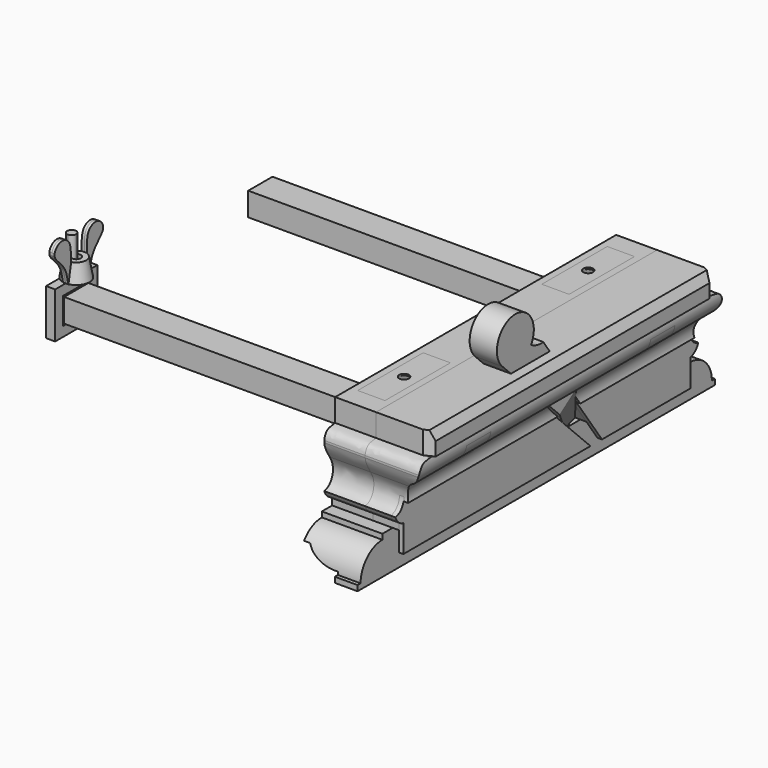
from build123d import *

# Parameters (mm, degrees)
F1_DEPTH  = 250
F2_DEPTH  = 250
F3_W      = 6.5
F3_H      = 13
F4_DEPTH  = 37.001
F8_DEPTH  = 15
F9_DEPTH  = 15
F10_W     = 20
F10_H     = 15.5
F11_DEPTH = 35.8337030046
F12_DEPTH = 50
F13_DEPTH = 230
F15_DEPTH = 20
F17_DEPTH = 20
F21_DEPTH = 9
F22_DEPTH = 27
F24_DEPTH = 40
F25_W     = 25
F25_H     = 3.6049708724
F26_DEPTH = 295.0010001
F27_DEPTH = 9
F29_REACH = 207.1008130873
F30_W     = 7
F30_H     = 35
F30_R     = 3.25
F31_DEPTH = 47
F30_W_2   = 18
F30_H_2   = 54
F32_DEPTH = 1
F33_DEPTH = 1
F34_DEPTH = 1
F35_W     = 22
F35_H     = 17.5
F36_DEPTH = 6
F37_R     = 2.99999
F39_DEPTH = 1.75


# Not quite as in the source:
# - a fillet or chamfer is up to 0.001 mm smaller than in the source, because OpenCascade refuses the exact size
# - a feature of the source that left no trace in its solid (it failed there, or was rolled back) is left out


with BuildPart() as f1:
    # F0 (on Front) → F1 (new body)
    with BuildSketch(Plane.XZ):
        with BuildLine():
            Line((0, 19.1666619313), (0, 0))
            Line((0, 0), (0, -42.8333380687))
            Line((0, -42.8333380687), (17, -42.8333380687))
            Line((17, -42.8333380687), (17, -22.8333380687))
            Line((17, -22.8333380687), (20, -22.8333380687))
            Line((20, -22.8333380687), (20, -25.2570672073))
            Line((20, -25.2570672073), (23, -25.2570672073))
            ThreePointArc((23, -25.2570672073), (23.5967218154, -16.8270536205), (29.25, -10.545202638))
            Line((29.25, -10.545202638), (35.5, 4.1666619313))
            Line((35.5, 4.1666619313), (37, 4.1666619313))
            Line((37, 4.1666619313), (37, 13.1666619313))
            Line((37, 13.1666619313), (34, 19.1666619313))
            Line((34, 19.1666619313), (0, 19.1666619313))
        make_face()
        with BuildLine():
            ThreePointArc((29.25, -10.545202638), (34.9032781846, -4.2633516555), (35.5, 4.1666619313))
            Line((35.5, 4.1666619313), (29.25, -10.545202638))
        make_face()
    extrude(amount=F1_DEPTH)


with BuildPart() as f2:
    # F0 (on Front) → F2 (new body)
    with BuildSketch(Plane.XZ):
        Polygon((17, -22.8333380687), (17, -42.8333380687), (17, -55.8333380687), (20, -55.8333380687), (20, -25.2570672073), (20, -22.8333380687), align=None)
    extrude(amount=F2_DEPTH)


with BuildPart() as f4_tool:
    # F3 (on face) → F4 (new body, through all)
    with BuildSketch(Plane(origin=(0, 0, 0), x_dir=(0, -1, 0), z_dir=(-1, 0, 0))):
        with BuildLine():
            Line((9, 4.1666619313), (9, 19.1666619313))
            Line((9, 19.1666619313), (0, 19.1666619313))
            Line((0, 19.1666619313), (0, -2.3163000296))
            add(Edge.make_bspline(
                [(9, 4.1666619313), (5.8723544835, 3.6611618628), (2.3380474739, 3.7477802491), (0.1732748267, -0.2324329033), (0, -2.3163000296)],
                knots=[0, 0, 0, 0, 0.1389392209, 0.2524518766, 0.2524518766, 0.2524518766, 0.2524518766], degree=3))
        make_face()
        with BuildLine():
            Line((250, 19.1666619313), (241, 19.1666619313))
            Line((241, 19.1666619313), (241, 4.1666619313))
            add(Edge.make_bspline(
                [(241, 4.1666619313), (244.1276455165, 3.6611618628), (247.6619525261, 3.7477802491), (249.8267251733, -0.2324329033), (250, -2.3163000296)],
                knots=[0, 0, 0, 0, 0.1389392209, 0.2524518766, 0.2524518766, 0.2524518766, 0.2524518766], degree=3))
            Line((250, -2.3163000296), (250, 19.1666619313))
        make_face()
        with BuildLine():
            add(Edge.make_bspline(
                [(4.5, -13.8333380687), (5.7822039131, -16.0114235416), (7.4274862503, -19.2486278619), (7.1721404656, -25.7962519699), (4.6179848399, -29.5292930366), (2.9422229886, -30.8853534567), (0.7419204277, -31.6729300915), (0, -31.8333380687)],
                knots=[0.4537350844, 0.4537350844, 0.4537350844, 0.4537350844, 0.5873526723, 0.7194908339, 0.8294393125, 0.9086679454, 1, 1, 1, 1], degree=3))
            Line((4.5, -13.8333380687), (0, -31.8333380687))
        make_face()
        with BuildLine():
            Line((0, -31.8333380687), (4.5, -13.8333380687))
            add(Edge.make_bspline(
                [(0, -3.6448843312), (0.283077162, -7.0636780394), (2.7941794565, -10.9356531472), (4.5, -13.8333380687)],
                knots=[0.2759726988, 0.2759726988, 0.2759726988, 0.2759726988, 0.4537350844, 0.4537350844, 0.4537350844, 0.4537350844], degree=3))
            Line((0, -3.6448843311), (0, -31.8333380687))
        make_face()
        with BuildLine():
            ThreePointArc((6.5, -37.8333380687), (2.4506727422, -35.6992759313), (0, -31.8333380687))
            Line((0, -31.8333380687), (0, -42.8333380687))
            Line((0, -42.8333380687), (6.5, -42.8333380687))
            Line((6.5, -42.8333380687), (6.5, -37.8333380687))
        make_face()
        with BuildLine():
            Line((250, -31.8333380687), (245.5, -13.8333380687))
            add(Edge.make_bspline(
                [(245.5, -13.8333380687), (244.2177960869, -16.0114235416), (242.5725137497, -19.2486278619), (242.8278595344, -25.7962519699), (245.3820151601, -29.5292930366), (247.0577770114, -30.8853534567), (249.2580795723, -31.6729300915), (250, -31.8333380687)],
                knots=[0.4537350844, 0.4537350844, 0.4537350844, 0.4537350844, 0.5873526723, 0.7194908339, 0.8294393125, 0.9086679454, 1, 1, 1, 1], degree=3))
        make_face()
        with BuildLine():
            add(Edge.make_bspline(
                [(250, -3.6448843312), (249.716922838, -7.0636780394), (247.2058205435, -10.9356531472), (245.5, -13.8333380687)],
                knots=[0.2759726988, 0.2759726988, 0.2759726988, 0.2759726988, 0.4537350844, 0.4537350844, 0.4537350844, 0.4537350844], degree=3))
            Line((245.5, -13.8333380687), (250, -31.8333380687))
            Line((250, -31.8333380687), (250, -3.6448843312))
        make_face()
        with Locations((3.25, -49.3333380687)):
            Rectangle(F3_W, F3_H)
        with BuildLine():
            Line((250, -42.8333380687), (250, -31.8333380687))
            ThreePointArc((250, -31.8333380687), (247.5493272578, -35.6992759313), (243.5, -37.8333380687))
            Line((243.5, -37.8333380687), (243.5, -42.8333380687))
            Line((243.5, -42.8333380687), (250, -42.8333380687))
        make_face()
        with Locations((246.75, -49.3333380687)):
            Rectangle(F3_W, F3_H)
    extrude(amount=-F4_DEPTH)


with BuildPart() as f1_1:
    add(f1.part)

    # F4: cut by f4_tool
    add(f4_tool.part, mode=Mode.SUBTRACT)

    # F7 (on face) → F8 (cut, through all)
    with BuildSketch(Plane.XY.offset(19.1666619313)):
        Polygon((34, -10.5), (34, -9), (31, -9), align=None)
        Polygon((37, -9), (34, -9), (34, -10.5), (37, -12), align=None)
    extrude(amount=-F8_DEPTH, mode=Mode.SUBTRACT)

    # F7 (on face) → F9 (cut, through all)
    with BuildSketch(Plane.XY.offset(19.1666619313)):
        Polygon((37, -238), (34, -239.5), (34, -241), (37, -241), align=None)
        Polygon((34, -241), (34, -239.5), (31, -241), align=None)
    extrude(amount=-F9_DEPTH, mode=Mode.SUBTRACT)

    # F10 (on face) → F11 (cut, through all)
    with BuildSketch(Plane(origin=(0, 0, 0), x_dir=(0, -1, 0), z_dir=(-1, 0, 0))):
        with Locations((49, -8.5833380687)):
            Rectangle(F10_W, F10_H)
        with Locations((201, -8.5833380687)):
            Rectangle(F10_W, F10_H)
    extrude(amount=-F11_DEPTH, mode=Mode.SUBTRACT)


with BuildPart() as f2_1:
    add(f2.part)

    # F4: cut by f4_tool
    add(f4_tool.part, mode=Mode.SUBTRACT)


with BuildPart() as f12:
    # F10 (on face) → F12 (new body)
    with BuildSketch(Plane(origin=(0, 0, 0), x_dir=(0, -1, 0), z_dir=(-1, 0, 0))):
        with Locations((201, -8.5833380687)):
            Rectangle(F10_W, F10_H)
    extrude(amount=-F12_DEPTH)

    # F10 (on face) → F13 (join)
    with BuildSketch(Plane(origin=(0, 0, 0), x_dir=(0, -1, 0), z_dir=(-1, 0, 0))):
        with Locations((201, -8.5833380687)):
            Rectangle(F10_W, F10_H)
    extrude(amount=F13_DEPTH)

    # F16 (on face) → F17 (cut, through all)
    with BuildSketch(Plane(origin=(0, -191, 0), x_dir=(-1, 0, 0), z_dir=(0, 1, 0))):
        with BuildLine():
            ThreePointArc((-23.8187110326, -16.3333380687), (-26.0817994285, -13.0146149671), (-29.25, -10.545202638))
            ThreePointArc((-29.25, -10.545202638), (-33.699272033, -6.474109032), (-35.8327030046, -0.8333380687))
            Line((-35.8327030046, -0.8333380687), (-50, -0.8333380687))
            Line((-50, -0.8333380687), (-50, -16.3333380687))
            Line((-50, -16.3333380687), (-23.8187110326, -16.3333380687))
        make_face()
    extrude(amount=-F17_DEPTH, mode=Mode.SUBTRACT)

    # F18: union 


with BuildPart() as f12b:
    # F10 (on face) → F12, piece 2 (new body)
    with BuildSketch(Plane(origin=(0, 0, 0), x_dir=(0, -1, 0), z_dir=(-1, 0, 0))):
        with Locations((49, -8.5833380687)):
            Rectangle(F10_W, F10_H)
    extrude(amount=-F12_DEPTH)

    # F10 (on face) → F13, piece 2 (join)
    with BuildSketch(Plane(origin=(0, 0, 0), x_dir=(0, -1, 0), z_dir=(-1, 0, 0))):
        with Locations((49, -8.5833380687)):
            Rectangle(F10_W, F10_H)
    extrude(amount=F13_DEPTH)

    # F14 (on face) → F15 (cut, through all)
    with BuildSketch(Plane(origin=(0, -39, 0), x_dir=(-1, 0, 0), z_dir=(0, 1, 0))):
        with BuildLine():
            ThreePointArc((-23.8187110326, -16.3333380686), (-26.0817994285, -13.0146149671), (-29.25, -10.545202638))
            ThreePointArc((-29.25, -10.545202638), (-33.699272033, -6.474109032), (-35.8327030046, -0.8333380687))
            Line((-35.8327030046, -0.8333380687), (-50, -0.8333380687))
            Line((-50, -0.8333380687), (-50, -16.3333380687))
            Line((-50, -16.3333380687), (-23.8187110326, -16.3333380687))
        make_face()
    extrude(amount=-F15_DEPTH, mode=Mode.SUBTRACT)


with BuildPart() as f21_tool:
    # F20 (on offset) → F21 (new body, symmetric)
    with BuildSketch(Plane(origin=(18.5, 0, 0), x_dir=(0, -1, 0), z_dir=(-1, 0, 0))):
        Polygon((102, -42.8333380687), (164, 19.1666619313), (132, 19.1666619313), (88.587132631, -42.8333380687), align=None)
        Polygon((89, -55.8333380687), (102, -42.8333380687), (88.587132631, -42.8333380687), (79.4844346343, -55.8333380687), align=None)
    extrude(amount=F21_DEPTH, both=True)


with BuildPart() as f1_2:
    add(f1_1.part)

    # F21: cut by f21_tool
    add(f21_tool.part, mode=Mode.SUBTRACT)


with BuildPart() as f2_2:
    add(f2_1.part)

    # F21: cut by f21_tool
    add(f21_tool.part, mode=Mode.SUBTRACT)


with BuildPart() as f22:
    # F22 (new): a face of the model
    f22_faces = [f1_2.part.faces().sort_by_distance(p)[0] for p in [
        (0, -125, -12.1189772339),
    ]]
    extrude(f22_faces, amount=F22_DEPTH)

    # F23 (on face) → F24 (join)
    with BuildSketch(Plane(origin=(-27, 0, 0), x_dir=(0, -1, 0), z_dir=(-1, 0, 0))):
        with BuildLine():
            Line((243.5, -42.8333380687), (6.5, -42.8333380687))
            Line((6.5, -42.8333380687), (-2, -42.8333380687))
            Line((-2, -42.8333380687), (-2, -46.3333380687))
            ThreePointArc((-2, -46.3333380687), (-14.7279220614, -51.6054160073), (-20, -64.3333380687))
            Line((-20, -64.3333380687), (-22.5, -64.3333380687))
            Line((-22.5, -64.3333380687), (-22.5, -67.9383089411))
            Line((-22.5, -67.9383089411), (272.5, -67.9383089411))
            Line((272.5, -67.9383089411), (272.5, -64.3333380687))
            Line((272.5, -64.3333380687), (270, -64.3333380687))
            ThreePointArc((270, -64.3333380687), (264.7279220614, -51.6054160073), (252, -46.3333380687))
            Line((252, -46.3333380687), (252, -42.8333380687))
            Line((252, -42.8333380687), (243.5, -42.8333380687))
        make_face()
    extrude(amount=-F24_DEPTH)

    # F25 (on face) → F26 (cut, through all)
    with BuildSketch(Plane(origin=(0, 22.5, 0), x_dir=(-1, 0, 0), z_dir=(0, 1, 0))):
        with BuildLine():
            Line((2, -62.4383089411), (2, -64.3333380687))
            Line((2, -64.3333380687), (27, -64.3333380687))
            Line((27, -64.3333380687), (27, -53.9383089411))
            Line((27, -53.9383089411), (23, -53.9383089411))
            ThreePointArc((23, -53.9383089411), (13.4744790698, -60.5958454666), (2, -62.4383089411))
        make_face()
        with Locations((14.5, -66.1358235049)):
            Rectangle(F25_W, F25_H)
    extrude(amount=-F26_DEPTH, mode=Mode.SUBTRACT)

    # F30 (on face) → F31 (cut)
    with BuildSketch(Plane.XY.offset(19.1666619313)):
        with Locations((-13.5, -49)):
            Rectangle(F30_W, F30_H)
        with Locations((-13.5, -49)):
            Circle(F30_R, mode=Mode.SUBTRACT)
        with Locations((-13.5, -201)):
            Rectangle(F30_W, F30_H)
        with Locations((-13.5, -201)):
            Circle(F30_R, mode=Mode.SUBTRACT)
        with Locations((-13.5, -49)):
            Circle(F30_R)
        with Locations((-13.5, -201)):
            Circle(F30_R)
    extrude(amount=-F31_DEPTH, mode=Mode.SUBTRACT)

    # F30 (on face) → F32 (cut)
    with BuildSketch(Plane.XY.offset(19.1666619313)):
        with Locations((-13.5, -201)):
            Rectangle(F30_W_2, F30_H_2)
        with Locations((-13.5, -201)):
            Rectangle(F30_W, F30_H, mode=Mode.SUBTRACT)
        with Locations((-13.5, -49)):
            Rectangle(F30_W_2, F30_H_2)
        with Locations((-13.5, -49)):
            Rectangle(F30_W, F30_H, mode=Mode.SUBTRACT)
    extrude(amount=-F32_DEPTH, mode=Mode.SUBTRACT)


with BuildPart() as f27:
    # F20 (on offset) → F27 (new body, symmetric)
    with BuildSketch(Plane(origin=(18.5, 0, 0), x_dir=(0, -1, 0), z_dir=(-1, 0, 0))):
        Polygon((102, -42.8333380687), (164, 19.1666619313), (132, 19.1666619313), (88.587132631, -42.8333380687), align=None)
        with BuildLine():
            Line((132, 19.1666619313), (164, 19.1666619313))
            Line((164, 19.1666619313), (171.1388857075, 26.3055476389))
            ThreePointArc((171.1388857075, 26.3055476389), (162.1789285126, 52.2079036357), (147.3491340876, 29.158173129))
            ThreePointArc((147.3491340876, 29.158173129), (142.5634500002, 27.0933830583), (137.3585397434, 26.8194497849))
            Line((137.3585397434, 26.8194497849), (132, 19.1666619313))
        make_face()
    extrude(amount=F27_DEPTH, both=True)

    f29_end = Plane(origin=(18.5, -136.5694428538, -8.2638952149), x_dir=(0, 0.7071067812, -0.7071067812), z_dir=(0, -0.7071067812, -0.7071067812))
    # F28 (on face) → F29 (cut, up to a plane its end follows)
    with BuildSketch(Plane(origin=(0, -79.5679440685, -55.7140742366), x_dir=(-1, 0, 0), z_dir=(0, 0.8191520443, 0.5735764364))):
        Polygon((-27.5, 15.7244753984), (-9.5, 15.7244753984), (-27.5, 53.7244753984), align=None)
    f29_long = extrude(amount=-F29_REACH, mode=Mode.PRIVATE)
    add(split(f29_long, bisect_by=f29_end, keep=Keep.BOTTOM, mode=Mode.PRIVATE), mode=Mode.SUBTRACT)


with BuildPart() as f33:
    # F30 (on face) → F33 (new body)
    with BuildSketch(Plane.XY.offset(19.1666619313)):
        with Locations((-13.5, -49)):
            Rectangle(F30_W_2, F30_H_2)
        with Locations((-13.5, -49)):
            Rectangle(F30_W, F30_H, mode=Mode.SUBTRACT)
        with Locations((-13.5, -49)):
            Rectangle(F30_W, F30_H)
        with Locations((-13.5, -49)):
            Circle(F30_R, mode=Mode.SUBTRACT)
    extrude(amount=-F33_DEPTH)


with BuildPart() as f34:
    # F30 (on face) → F34 (new body)
    with BuildSketch(Plane.XY.offset(19.1666619313)):
        with Locations((-13.5, -201)):
            Rectangle(F30_W_2, F30_H_2)
        with Locations((-13.5, -201)):
            Rectangle(F30_W, F30_H, mode=Mode.SUBTRACT)
        with Locations((-13.5, -201)):
            Rectangle(F30_W, F30_H)
        with Locations((-13.5, -201)):
            Circle(F30_R, mode=Mode.SUBTRACT)
    extrude(amount=-F34_DEPTH)


with BuildPart() as f36:
    # F35 (on face) → F36 (new body)
    with BuildSketch(Plane(origin=(-230, 0, 0), x_dir=(0, -1, 0), z_dir=(-1, 0, 0))):
        Polygon((218.4000015259, -23.7333395945), (218.4000015259, 6.5666634572), (209.75, 6.5666634572), (204, 6.5666634572), (204, 18.5666634572), (204, 31.5666634572), (198, 31.5666634572), (198, 18.5666634572), (198, 6.5666634572), (192.25, 6.5666634572), (183.5999984741, 6.5666634572), (183.5999984741, -23.7333395945), align=None)
        with Locations((201, -8.5833380687)):
            Rectangle(F35_W, F35_H, mode=Mode.SUBTRACT)
    extrude(amount=F36_DEPTH)

    # F37 (radius 3 in the source; OpenCascade refuses exactly that, so slightly less here)
    f37_edges = [f36.edges().sort_by_distance(p)[0] for p in [
        (-236, -204, 19.066663),
        (-230, -204, 19.066663),
        (-236, -198, 19.066663),
        (-230, -198, 19.066663),
    ]]
    fillet(f37_edges, radius=F37_R)


with BuildPart() as f38:
    # F35 (on face) → F38 (revolve)
    with BuildSketch(Plane(origin=(-230, 0, 0), x_dir=(0, -1, 0), z_dir=(-1, 0, 0))):
        Polygon((204, 6.5666634572), (209.75, 6.5666634572), (207.633645577, 18.5666634572), (204, 18.5666634572), align=None)
    revolve(axis=Axis((-230, -201, 17.2606460741), (0, 0, 1)))

    # F35 (on face) → F39 (join, symmetric)
    with BuildSketch(Plane(origin=(-230, 0, 0), x_dir=(0, -1, 0), z_dir=(-1, 0, 0))):
        Polygon((204, 6.5666634572), (209.75, 6.5666634572), (207.633645577, 18.5666634572), (204, 18.5666634572), align=None)
        with BuildLine():
            Line((207.633645577, 18.5666634572), (209.75, 6.5666634572))
            add(Edge.make_bspline(
                [(221, 27.3085609078), (220.5142732506, 25.0966716249), (215.471671147, 20.8693652085), (211.378546536, 15.0964185722), (210.5969494366, 10.5985070963), (209.75, 6.5666634572)],
                knots=[0.6040363988, 0.6040363988, 0.6040363988, 0.6040363988, 0.7384341166, 0.8605009012, 1, 1, 1, 1], degree=3))
            Line((221, 27.3085609078), (221, 28.9294647519))
            add(Edge.make_bspline(
                [(207.633645577, 18.5666634572), (207.5657790254, 19.4166297823), (207.7027476853, 21.5795836916), (207.5384260425, 30.4438036433), (212.3834660875, 33.7615072096), (216.1214157744, 33.9970320723), (219.2832722056, 32.387319528), (220.7750000105, 30.0256084268), (221, 28.9294647519)],
                knots=[0, 0, 0, 0, 0.080789482, 0.2163324063, 0.3233343812, 0.4105273732, 0.5018531212, 0.5708228321, 0.5708228321, 0.5708228321, 0.5708228321], degree=3))
        make_face()
        Polygon((194.366354423, 18.5666634572), (192.25, 6.5666634572), (198, 6.5666634572), (198, 18.5666634572), align=None)
        with BuildLine():
            add(Edge.make_bspline(
                [(194.366354423, 18.5666634572), (194.4342209746, 19.4166297823), (194.2972523147, 21.5795836916), (194.4615739575, 30.4438036433), (189.6165339125, 33.7615072096), (185.8785842256, 33.9970320723), (182.292398784, 32.1712920942), (179.4766003172, 26.7809593961), (186.528328853, 20.8693652085), (190.621453464, 15.0964185722), (191.4030505634, 10.5985070963), (192.25, 6.5666634572)],
                knots=[0, 0, 0, 0, 0.080789482, 0.2163324063, 0.3233343812, 0.4105273732, 0.5018531212, 0.6040363988, 0.7384341166, 0.8605009012, 1, 1, 1, 1], degree=3))
            Line((192.25, 6.5666634572), (194.366354423, 18.5666634572))
        make_face()
    extrude(amount=F39_DEPTH, both=True)


solid = Compound([f12.part, f12b.part, f1_2.part, f2_2.part, f22.part, f27.part, f33.part, f34.part, f36.part, f38.part])
